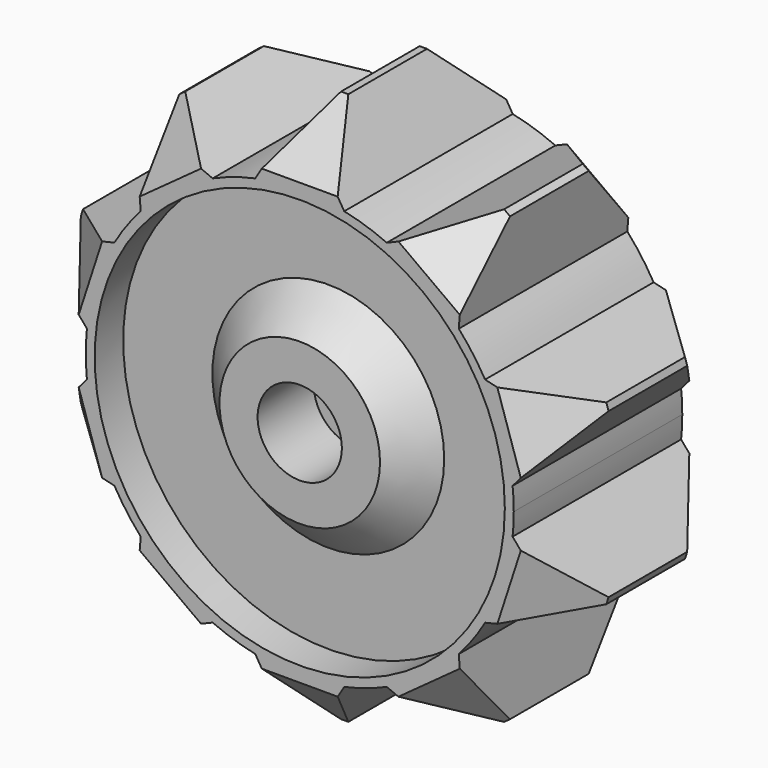
from build123d import *

# Parameters (mm, degrees)
F1_DEPTH = 15
F2_SIZE  = 0.5
F3_SIZE  = 4
F4_R     = 2
F5_DEPTH = 25.4
F6_R     = 3
F7_DEPTH = 5
F8_R     = 14.605
F8_R_2   = 3.175
F9_DEPTH = 2.54


# Not quite as in the source:
# - a fillet or chamfer that OpenCascade refuses, or shapes differently, is made with other operations: its cross-section is extruded or revolved along the edge and cut away or added


with BuildPart() as f1:
    # F0 (on Front) → F1 (new body)
    with BuildSketch(Plane.XZ):
        with BuildLine():
            Line((0, -20.1), (3.1676147888, -14.9071733253))
            ThreePointArc((3.1676147888, -14.9071733253), (0, -15.24), (-3.1676147888, -14.9071733253))
            Line((-3.1676147888, -14.9071733253), (0, -20.1))
        make_face()
        with BuildLine():
            ThreePointArc((-3.1676147888, 14.9071733253), (0, 15.24), (3.1676147888, 14.9071733253))
            Line((3.1676147888, 14.9071733253), (0, 20.1))
            Line((0, 20.1), (-3.1676147888, 14.9071733253))
        make_face()
        with BuildLine():
            ThreePointArc((-11.3248708297, 10.1982793004), (-8.9578472449, 12.3294189943), (-6.1995624382, 13.922033816))
            Line((-6.1995624382, 13.922033816), (-11.8144835711, 16.2612415869))
            Line((-11.8144835711, 16.2612415869), (-11.3248708297, 10.1982793004))
        make_face()
        with BuildLine():
            ThreePointArc((-15.1564111319, 1.5939892096), (-14.4941013083, 4.7094189943), (-13.1987175292, 7.6191505816))
            Line((-13.1987175292, 7.6191505816), (-19.1162359775, 6.2112415869))
            Line((-19.1162359775, 6.2112415869), (-15.1564111319, 1.5939892096))
        make_face()
        with BuildLine():
            Line((-19.1162359775, -6.2112415869), (-13.1987175292, -7.6191505816))
            ThreePointArc((-13.1987175292, -7.6191505816), (-14.4941013083, -4.7094189943), (-15.1564111319, -1.5939892096))
            Line((-15.1564111319, -1.5939892096), (-19.1162359775, -6.2112415869))
        make_face()
        with BuildLine():
            Line((-11.8144835711, -16.2612415869), (-6.1995624382, -13.922033816))
            ThreePointArc((-6.1995624382, -13.922033816), (-8.9578472449, -12.3294189943), (-11.3248708297, -10.1982793004))
            Line((-11.3248708297, -10.1982793004), (-11.8144835711, -16.2612415869))
        make_face()
        with BuildLine():
            ThreePointArc((15.1564111319, -1.5939892096), (15.2190884361, -0.7980897035), (15.24, 0))
            ThreePointArc((15.24, 0), (15.2190884361, 0.7980897035), (15.1564111319, 1.5939892096))
            ThreePointArc((15.1564111319, 1.5939892096), (14.4941013083, 4.7094189943), (13.1987175292, 7.6191505816))
            ThreePointArc((13.1987175292, 7.6191505816), (12.3294189943, 8.9578472449), (11.3248708297, 10.1982793004))
            ThreePointArc((11.3248708297, 10.1982793004), (8.9578472449, 12.3294189943), (6.1995624382, 13.922033816))
            ThreePointArc((6.1995624382, 13.922033816), (4.7094189943, 14.4941013083), (3.1676147888, 14.9071733253))
            ThreePointArc((3.1676147888, 14.9071733253), (0, 15.24), (-3.1676147888, 14.9071733253))
            ThreePointArc((-3.1676147888, 14.9071733253), (-4.7094189943, 14.4941013083), (-6.1995624382, 13.922033816))
            ThreePointArc((-6.1995624382, 13.922033816), (-8.9578472449, 12.3294189943), (-11.3248708297, 10.1982793004))
            ThreePointArc((-11.3248708297, 10.1982793004), (-12.3294189943, 8.9578472449), (-13.1987175292, 7.6191505816))
            ThreePointArc((-13.1987175292, 7.6191505816), (-14.4941013083, 4.7094189943), (-15.1564111319, 1.5939892096))
            ThreePointArc((-15.1564111319, 1.5939892096), (-15.24, 0), (-15.1564111319, -1.5939892096))
            ThreePointArc((-15.1564111319, -1.5939892096), (-14.4941013083, -4.7094189943), (-13.1987175292, -7.6191505816))
            ThreePointArc((-13.1987175292, -7.6191505816), (-12.3294189943, -8.9578472449), (-11.3248708297, -10.1982793004))
            ThreePointArc((-11.3248708297, -10.1982793004), (-8.9578472449, -12.3294189943), (-6.1995624382, -13.922033816))
            ThreePointArc((-6.1995624382, -13.922033816), (-4.7094189943, -14.4941013083), (-3.1676147888, -14.9071733253))
            ThreePointArc((-3.1676147888, -14.9071733253), (0, -15.24), (3.1676147888, -14.9071733253))
            ThreePointArc((3.1676147888, -14.9071733253), (4.7094189943, -14.4941013083), (6.1995624382, -13.922033816))
            ThreePointArc((6.1995624382, -13.922033816), (8.9578472449, -12.3294189943), (11.3248708297, -10.1982793004))
            ThreePointArc((11.3248708297, -10.1982793004), (12.3294189943, -8.9578472449), (13.1987175292, -7.6191505816))
            ThreePointArc((13.1987175292, -7.6191505816), (14.4941013083, -4.7094189943), (15.1564111319, -1.5939892096))
        make_face()
        with BuildLine():
            ThreePointArc((6.1995624382, 13.922033816), (8.9578472449, 12.3294189943), (11.3248708297, 10.1982793004))
            Line((11.3248708297, 10.1982793004), (11.8144835711, 16.2612415869))
            Line((11.8144835711, 16.2612415869), (6.1995624382, 13.922033816))
        make_face()
        with BuildLine():
            ThreePointArc((13.1987175292, 7.6191505816), (14.4941013083, 4.7094189943), (15.1564111319, 1.5939892096))
            Line((15.1564111319, 1.5939892096), (19.1162359775, 6.2112415869))
            Line((19.1162359775, 6.2112415869), (13.1987175292, 7.6191505816))
        make_face()
        with BuildLine():
            Line((19.1162359775, -6.2112415869), (15.1564111319, -1.5939892096))
            ThreePointArc((15.1564111319, -1.5939892096), (14.4941013083, -4.7094189943), (13.1987175292, -7.6191505816))
            Line((13.1987175292, -7.6191505816), (19.1162359775, -6.2112415869))
        make_face()
        with BuildLine():
            Line((11.8144835711, -16.2612415869), (11.3248708297, -10.1982793004))
            ThreePointArc((11.3248708297, -10.1982793004), (8.9578472449, -12.3294189943), (6.1995624382, -13.922033816))
            Line((6.1995624382, -13.922033816), (11.8144835711, -16.2612415869))
        make_face()
    extrude(amount=F1_DEPTH)

    # F2
    f2_edges = [f1.edges().sort_by_distance(p)[0] for p in [
        (0, -7.5, -20.1),
        (0, -7.5, 20.1),
        (-11.814484, -7.5, -16.261242),
        (-19.116236, -7.5, -6.211242),
        (-19.116236, -7.5, 6.211242),
        (-11.814484, -7.5, 16.261242),
        (11.814484, -7.5, 16.261242),
        (19.116236, -7.5, 6.211242),
        (19.116236, -7.5, -6.211242),
        (11.814484, -7.5, -16.261242),
    ]]
    chamfer(f2_edges, length=F2_SIZE)

    # F3
    f3_edges = [f1.edges().sort_by_distance(p)[0] for p in [
        (-11.563586, -15, 15.915911),
        (-11.563586, 0, 15.915911),
        (0, 0, 19.673148),
        (0, -15, 19.673148),
        (0, -15, -19.673148),
        (-11.563586, -15, -15.915911),
        (-18.710275, -15, -6.079337),
        (-18.710275, -15, 6.079337),
        (-18.710275, 0, 6.079337),
        (-18.710275, 0, -6.079337),
        (-11.563586, 0, -15.915911),
        (0, 0, -19.673148),
        (11.563586, -15, 15.915911),
        (18.710275, -15, 6.079337),
        (18.710275, -15, -6.079337),
        (11.563586, -15, -15.915911),
        (11.563586, 0, 15.915911),
        (18.710275, 0, 6.079337),
        (18.710275, 0, -6.079337),
        (11.563586, 0, -15.915911),
    ]]
    chamfer(f3_edges, length=F3_SIZE)

    # F4 (on face) → F5 (cut)
    with BuildSketch(Plane.XZ.offset(15)):
        Circle(F4_R)
    extrude(amount=-F5_DEPTH, mode=Mode.SUBTRACT)

    # F6 (on face) → F7 (cut)
    with BuildSketch(Plane.XZ.offset(15)):
        Circle(F6_R)
    extrude(amount=-F7_DEPTH, mode=Mode.SUBTRACT)

    # F8 (on face) → F9 (cut)
    with BuildSketch(Plane.XZ.offset(15)):
        Circle(F8_R)
        Circle(F8_R_2, mode=Mode.SUBTRACT)
    extrude(amount=-F9_DEPTH, mode=Mode.SUBTRACT)

    # F10: chamfer of 5.08 on 1 edges, made by hand


with BuildPart() as f10_tool2:
    # F10_s3 → F10_t4 (revolve)
    with BuildSketch(Plane.XY):
        Polygon((8.255, -12.46), (3.175, -17.54), (3.175, -12.46), align=None)
    revolve(axis=Axis((0, -12.46, 0), (0, -1, 0)))

    split(bisect_by=Plane.XZ.offset(15), keep=Keep.BOTTOM)


with BuildPart() as f1_1:
    add(f1.part)

    # F10_t1: union F10_tool2
    add(f10_tool2.part)


solid = f1_1.part
